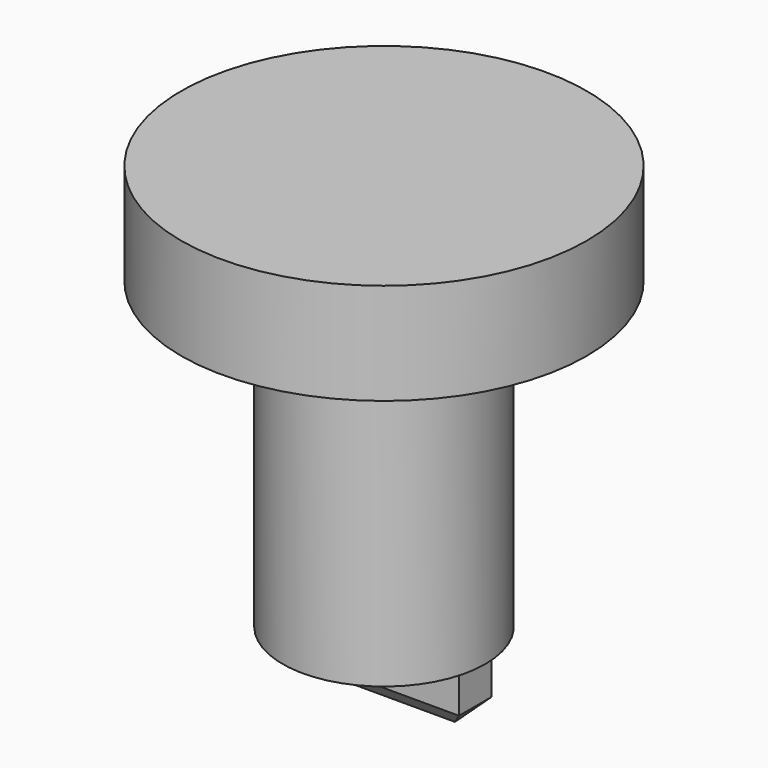
from build123d import *

# Parameters (mm, degrees)
F0_R     = 10
F1_DEPTH = 5
F2_R     = 5
F3_DEPTH = 15
F4_W     = 9
F4_H     = 2
F5_DEPTH = 3
F6_SIZE  = 0.99999


# Not quite as in the source:
# - a fillet or chamfer is up to 0.001 mm smaller than in the source, because OpenCascade refuses the exact size


with BuildPart() as f1:
    # F0 (on Top) → F1 (new body)
    with BuildSketch(Plane.XY):
        Circle(F0_R)
    extrude(amount=-F1_DEPTH)

    # F2 (on face) → F3 (join)
    with BuildSketch(Plane(origin=(0, 0, -5), x_dir=(1, 0, 0), z_dir=(0, 0, -1))):
        Circle(F2_R)
    extrude(amount=F3_DEPTH)

    # F4 (on face) → F5 (join)
    with BuildSketch(Plane(origin=(0, 0, -20), x_dir=(1, 0, 0), z_dir=(0, 0, -1))):
        Rectangle(F4_W, F4_H)
    extrude(amount=F5_DEPTH)

    # F6 (size 1 in the source; OpenCascade refuses exactly that, so slightly less here)
    f6_edges = [f1.edges().sort_by_distance(p)[0] for p in [
        (0, -1, -23),
        (-4.5, 0, -23),
        (0, 1, -23),
        (4.5, 0, -23),
    ]]
    chamfer(f6_edges, length=F6_SIZE)


solid = f1.part
